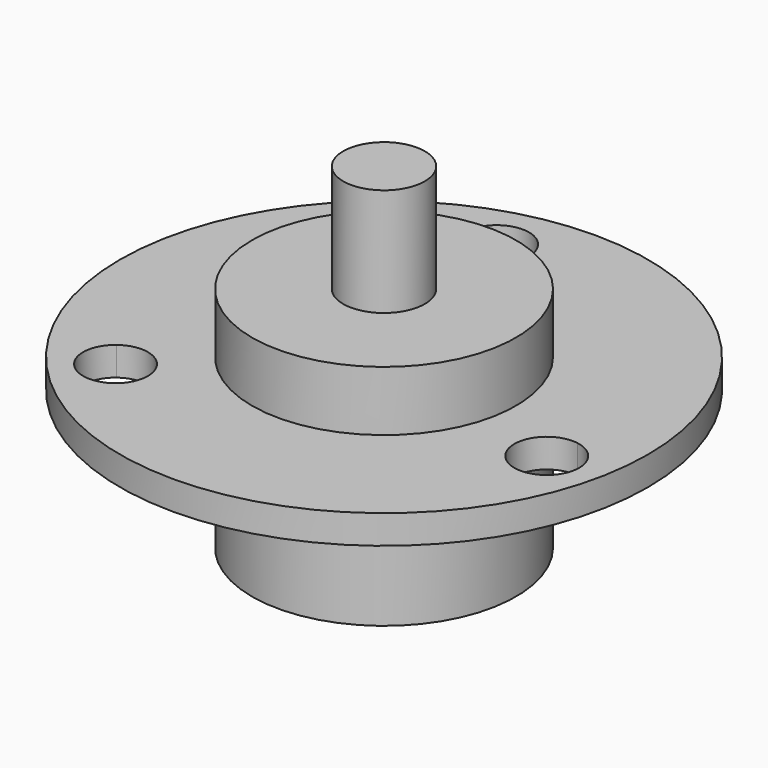
from build123d import *

# Parameters (mm, degrees)
F3_DEPTH = 2.4


with BuildPart() as f1:
    # F0 (on Front) → F1 (revolve)
    with BuildSketch(Plane.XZ):
        Polygon((-130.5134040415, -110.4772146098), (-130.5134040415, -122.0772146098), (-119.5134040415, -122.0772146098), (-119.5134040415, -94.0772146098), (-122.9134040415, -94.0772146098), (-122.9134040415, -103.0772146098), (-130.5134040415, -103.0772146098), (-130.5134040415, -108.0772146098), (-141.5134040415, -108.0772146098), (-141.5134040415, -110.4772146098), align=None)
    revolve(axis=Axis((-119.5134040415, 0, -108.0772146098), (0, 0, -1)))

    # F2 (on face) → F3 (cut, through all)
    with BuildSketch(Plane.XY.offset(-108.0772146098)):
        with BuildLine():
            ThreePointArc((-121.0167680789, 16.9876935094), (-121.0259896486, 17.2106541317), (-121.0535913671, 17.4320917564))
            ThreePointArc((-121.0535913671, 17.4320917564), (-123.7167680789, 16.9876935094), (-126.27988757, 16.1389188194))
            ThreePointArc((-126.27988757, 16.1389188194), (-123.2868975321, 14.3221332844), (-121.0167680789, 16.9876935094))
        make_face()
        with BuildLine():
            ThreePointArc((-126.27988757, 16.1389188194), (-123.7167680789, 16.9876935094), (-121.0535913671, 17.4320917564))
            ThreePointArc((-121.0535913671, 17.4320917564), (-124.3652871018, 19.6086519366), (-126.27988757, 16.1389188194))
        make_face()
        with BuildLine():
            ThreePointArc((-99.8403964321, -4.2622778759), (-100.4770477105, -2.5208439688), (-102.0867609158, -1.6006590418))
            ThreePointArc((-102.0867609158, -1.6006590418), (-102.5403964321, -4.2622778759), (-103.3980588072, -6.8224370996))
            ThreePointArc((-103.3980588072, -6.8224370996), (-100.9633245271, -6.4538171082), (-99.8403964321, -4.2622778759))
        make_face()
        with BuildLine():
            ThreePointArc((-103.3980588072, -6.8224370996), (-102.5403964321, -4.2622778759), (-102.0867609158, -1.6006590418))
            ThreePointArc((-102.0867609158, -1.6006590418), (-105.1590890347, -3.6046692894), (-103.3980588072, -6.8224370996))
        make_face()
        with BuildLine():
            ThreePointArc((-129.8403964321, -11.6853527655), (-131.3455427368, -9.2641289744), (-134.1828591335, -9.5423837329))
            ThreePointArc((-134.1828591335, -9.5423837329), (-132.5403964321, -11.6853527655), (-130.5878381405, -13.550162707))
            ThreePointArc((-130.5878381405, -13.550162707), (-130.0342133395, -12.6898657352), (-129.8403964321, -11.6853527655))
        make_face()
        with BuildLine():
            ThreePointArc((-130.5878381405, -13.550162707), (-132.5403964321, -11.6853527655), (-134.1828591335, -9.5423837329))
            ThreePointArc((-134.1828591335, -9.5423837329), (-134.5502752581, -13.4882357636), (-130.5878381405, -13.550162707))
        make_face()
    extrude(amount=-F3_DEPTH, mode=Mode.SUBTRACT)


solid = f1.part
